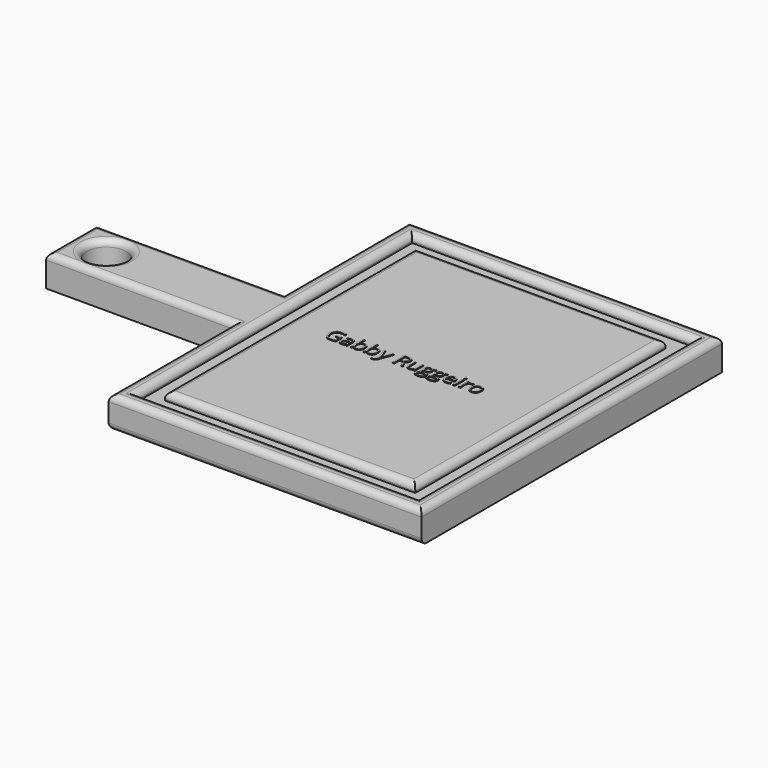
from build123d import *

# Parameters (mm, degrees)
F0_W         = 152.4
F0_H         = 50.8
F1_DEPTH     = 25.4
F2_R         = 15.875
F3_DEPTH     = 25.4
F5_DEPTH     = 6.35
F6_T1_DEPTH  = 228.5999910355
F6_T3_DEPTH  = 279.3999910355
F6_T5_DEPTH  = 330.2
F6_T7_DEPTH  = 279.4
F6_T9_DEPTH  = 139.7
F6_T11_DEPTH = 139.7
F6_T13_DEPTH = 228.5999783039
F6_T15_DEPTH = 279.3999783039
F6_T17_DEPTH = 76.2
F6_T19_DEPTH = 165.1
F6_T27_DEPTH = 292.0999910355
F6_T31_DEPTH = 241.2999910355
F6_T38_DEPTH = 241.2999910355
F6_T42_DEPTH = 292.0999910355
F6_T49_DEPTH = 292.0999910355
F6_T53_DEPTH = 241.2999910355
F6_T60_DEPTH = 292.0999910355
F6_T64_DEPTH = 241.2999910355
F6_T71_DEPTH = 152.4
F6_T75_DEPTH = 177.8
F6_T82_DEPTH = 152.4
F6_T86_DEPTH = 177.8
F7_TEXT_SIZE = 17.0792183232
F8_DEPTH     = 0.508


# Not quite as in the source:
# - a fillet or chamfer that OpenCascade refuses, or shapes differently, is made with other operations: its cross-section is extruded or revolved along the edge and cut away or added
# - Text() gives the source's letters only with a copy of the font that has no kerning and outlines rounded to 1/6400 em; it was checked with that copy


with BuildPart() as f1:
    # F0 (on Top) → F1 (new body)
    with BuildSketch(Plane.XY):
        Polygon((127, -152.4), (127, 152.4), (-127, 152.4), (-127, 25.4), (-127, -25.4), (-127, -152.4), align=None)
        with Locations((-203.2, 0)):
            Rectangle(F0_W, F0_H)
    extrude(amount=F1_DEPTH)

    # F2 (on face) → F3 (cut)
    with BuildSketch(Plane.XY.offset(25.4)):
        with Locations((-250.825, 0)):
            Circle(F2_R)
    extrude(amount=-F3_DEPTH, mode=Mode.SUBTRACT)

    # F4 (on face) → F5 (cut)
    with BuildSketch(Plane.XY.offset(25.4)):
        Polygon((114.2999955177, 139.6999955177), (-114.2999955177, 139.6999955177), (-114.2999955177, 25.4), (-114.2999955177, -25.4), (-114.2999955177, -139.6999955177), (114.2999955177, -139.6999955177), align=None)
        Polygon((-101.599989152, 126.999989152), (101.599989152, 126.999989152), (101.599989152, -126.999989152), (-101.599989152, -126.999989152), (-101.599989152, -25.4), (-101.599989152, 25.4), align=None, mode=Mode.SUBTRACT)
    extrude(amount=-F5_DEPTH, mode=Mode.SUBTRACT)

    # F6: fillet of radius 5.08 on 19 edges, made by hand

    # F6_s2 → F6_t1 (cut)
    with BuildSketch(Plane.YZ.offset(-114.2999955177)):
        with BuildLine():
            ThreePointArc((144.7799955177, 25.4), (141.1878930693, 23.9121024484), (139.6999955177, 20.32))
            Line((139.6999955177, 20.32), (139.6999955177, 25.4))
            Line((139.6999955177, 25.4), (144.7799955177, 25.4))
        make_face()
        with BuildLine():
            ThreePointArc((-144.7799955177, 25.4), (-141.1878930693, 23.9121024484), (-139.6999955177, 20.32))
            Line((-139.6999955177, 20.32), (-139.6999955177, 25.4))
            Line((-139.6999955177, 25.4), (-144.7799955177, 25.4))
        make_face()
    extrude(amount=F6_T1_DEPTH, mode=Mode.SUBTRACT)

    # F6_s4 → F6_t3 (cut)
    with BuildSketch(Plane.XZ.offset(-139.6999955177)):
        with BuildLine():
            ThreePointArc((-119.3799955177, 25.4), (-115.7878930693, 23.9121024484), (-114.2999955177, 20.32))
            Line((-114.2999955177, 20.32), (-114.2999955177, 25.4))
            Line((-114.2999955177, 25.4), (-119.3799955177, 25.4))
        make_face()
        with BuildLine():
            ThreePointArc((119.3799955177, 25.4), (115.7878930693, 23.9121024484), (114.2999955177, 20.32))
            Line((114.2999955177, 20.32), (114.2999955177, 25.4))
            Line((114.2999955177, 25.4), (119.3799955177, 25.4))
        make_face()
    extrude(amount=F6_T3_DEPTH, mode=Mode.SUBTRACT)

    # F6_s6 → F6_t5 (cut)
    with BuildSketch(Plane.XZ.offset(-165.1)):
        with BuildLine():
            ThreePointArc((127, 20.32), (125.5121024484, 23.9121024484), (121.92, 25.4))
            Line((121.92, 25.4), (127, 25.4))
            Line((127, 25.4), (127, 20.32))
        make_face()
    extrude(amount=F6_T5_DEPTH, mode=Mode.SUBTRACT)

    # F6_s8 → F6_t7 (cut)
    with BuildSketch(Plane.YZ.offset(-139.7)):
        with BuildLine():
            ThreePointArc((-152.4, 20.32), (-150.9121024484, 23.9121024484), (-147.32, 25.4))
            Line((-147.32, 25.4), (-152.4, 25.4))
            Line((-152.4, 25.4), (-152.4, 20.32))
        make_face()
        with BuildLine():
            ThreePointArc((152.4, 20.32), (150.9121024484, 23.9121024484), (147.32, 25.4))
            Line((147.32, 25.4), (152.4, 25.4))
            Line((152.4, 25.4), (152.4, 20.32))
        make_face()
        with BuildLine():
            ThreePointArc((-152.4, 5.08), (-150.9121024484, 1.4878975516), (-147.32, 0))
            Line((-147.32, 0), (-152.4, 0))
            Line((-152.4, 0), (-152.4, 5.08))
        make_face()
    extrude(amount=F6_T7_DEPTH, mode=Mode.SUBTRACT)

    # F6_s10 → F6_t9 (cut)
    with BuildSketch(Plane.XZ.offset(25.4)):
        with BuildLine():
            ThreePointArc((-121.92, 25.4), (-125.5121024484, 23.9121024484), (-127, 20.32))
            Line((-127, 20.32), (-127, 25.4))
            Line((-127, 25.4), (-121.92, 25.4))
        make_face()
        with BuildLine():
            ThreePointArc((-121.92, 0), (-125.5121024484, 1.4878975516), (-127, 5.08))
            Line((-127, 5.08), (-127, 0))
            Line((-127, 0), (-121.92, 0))
        make_face()
    extrude(amount=F6_T9_DEPTH, mode=Mode.SUBTRACT)

    # F6_s12 → F6_t11 (cut)
    with BuildSketch(Plane.XZ.offset(-165.1)):
        with BuildLine():
            ThreePointArc((-121.92, 25.4), (-125.5121024484, 23.9121024484), (-127, 20.32))
            Line((-127, 20.32), (-127, 25.4))
            Line((-127, 25.4), (-121.92, 25.4))
        make_face()
    extrude(amount=F6_T11_DEPTH, mode=Mode.SUBTRACT)

    # F6_s14 → F6_t13 (cut)
    with BuildSketch(Plane.YZ.offset(-114.299989152)):
        with BuildLine():
            ThreePointArc((126.999989152, 20.32), (125.5120916004, 23.9121024484), (121.919989152, 25.4))
            Line((121.919989152, 25.4), (126.999989152, 25.4))
            Line((126.999989152, 25.4), (126.999989152, 20.32))
        make_face()
        with BuildLine():
            ThreePointArc((-126.999989152, 20.32), (-125.5120916004, 23.9121024484), (-121.919989152, 25.4))
            Line((-121.919989152, 25.4), (-126.999989152, 25.4))
            Line((-126.999989152, 25.4), (-126.999989152, 20.32))
        make_face()
    extrude(amount=F6_T13_DEPTH, mode=Mode.SUBTRACT)

    # F6_s16 → F6_t15 (cut)
    with BuildSketch(Plane.XZ.offset(-139.699989152)):
        with BuildLine():
            ThreePointArc((101.599989152, 20.32), (100.1120916004, 23.9121024484), (96.519989152, 25.4))
            Line((96.519989152, 25.4), (101.599989152, 25.4))
            Line((101.599989152, 25.4), (101.599989152, 20.32))
        make_face()
        with BuildLine():
            ThreePointArc((-101.599989152, 20.32), (-100.1120916004, 23.9121024484), (-96.519989152, 25.4))
            Line((-96.519989152, 25.4), (-101.599989152, 25.4))
            Line((-101.599989152, 25.4), (-101.599989152, 20.32))
        make_face()
    extrude(amount=F6_T15_DEPTH, mode=Mode.SUBTRACT)

    # F6_s18 → F6_t17 (cut)
    with BuildSketch(Plane.XZ.offset(-38.1)):
        with BuildLine():
            ThreePointArc((-274.32, 25.4), (-277.9121024484, 23.9121024484), (-279.4, 20.32))
            Line((-279.4, 20.32), (-279.4, 25.4))
            Line((-279.4, 25.4), (-274.32, 25.4))
        make_face()
    extrude(amount=F6_T17_DEPTH, mode=Mode.SUBTRACT)

    # F6_s20 → F6_t19 (cut)
    with BuildSketch(Plane.YZ.offset(-292.1)):
        with BuildLine():
            ThreePointArc((20.32, 25.4), (23.9121024484, 23.9121024484), (25.4, 20.32))
            Line((25.4, 20.32), (25.4, 25.4))
            Line((25.4, 25.4), (20.32, 25.4))
        make_face()
        with BuildLine():
            ThreePointArc((-20.32, 25.4), (-23.9121024484, 23.9121024484), (-25.4, 20.32))
            Line((-25.4, 20.32), (-25.4, 25.4))
            Line((-25.4, 25.4), (-20.32, 25.4))
        make_face()
    extrude(amount=F6_T19_DEPTH, mode=Mode.SUBTRACT)

    # F6_s21 → F6_t22 (revolve, cut)
    with BuildSketch(Plane.XZ):
        with BuildLine():
            ThreePointArc((-229.87, 25.4), (-233.4621024484, 23.9121024484), (-234.95, 20.32))
            Line((-234.95, 20.32), (-234.95, 25.4))
            Line((-234.95, 25.4), (-229.87, 25.4))
        make_face()
    revolve(axis=Axis((-250.825, 0, 25.4), (0, 0, 1)), mode=Mode.SUBTRACT)


with BuildPart() as f6_tool25:
    # F6_s26 → F6_t27 (new body)
    with BuildSketch(Plane.XZ.offset(139.6999955177)):
        with BuildLine():
            ThreePointArc((119.3799955177, 25.4), (115.7878930693, 23.9121024484), (114.2999955177, 20.32))
            Line((114.2999955177, 20.32), (114.2999955177, 25.4))
            Line((114.2999955177, 25.4), (119.3799955177, 25.4))
        make_face()
    extrude(amount=-F6_T27_DEPTH)

    split(bisect_by=Plane.XZ.offset(-139.6999955177), keep=Keep.BOTTOM)


with BuildPart() as f6_tool29:
    # F6_s30 → F6_t31 (new body)
    with BuildSketch(Plane.YZ.offset(126.9999955177)):
        with BuildLine():
            ThreePointArc((144.7799955177, 25.4), (141.1878930693, 23.9121024484), (139.6999955177, 20.32))
            Line((139.6999955177, 20.32), (139.6999955177, 25.4))
            Line((139.6999955177, 25.4), (144.7799955177, 25.4))
        make_face()
    extrude(amount=-F6_T31_DEPTH)

    split(bisect_by=Plane.YZ.offset(114.2999955177), keep=Keep.TOP)


with BuildPart() as f6_tool25_1:
    add(f6_tool25.part)

    # F6_t33: intersect F6_tool29
    add(f6_tool29.part, mode=Mode.INTERSECT)


with BuildPart() as f1_1:
    add(f1.part)

    # F6_t23: cut F6_tool25
    add(f6_tool25_1.part, mode=Mode.SUBTRACT)


with BuildPart() as f6_tool36:
    # F6_s37 → F6_t38 (new body)
    with BuildSketch(Plane.YZ.offset(114.2999955177)):
        with BuildLine():
            ThreePointArc((144.7799955177, 25.4), (141.1878930693, 23.9121024484), (139.6999955177, 20.32))
            Line((139.6999955177, 20.32), (139.6999955177, 25.4))
            Line((139.6999955177, 25.4), (144.7799955177, 25.4))
        make_face()
    extrude(amount=-F6_T38_DEPTH)

    split(bisect_by=Plane.YZ.offset(-114.2999955177), keep=Keep.BOTTOM)


with BuildPart() as f6_tool40:
    # F6_s41 → F6_t42 (new body)
    with BuildSketch(Plane.XZ.offset(139.6999955177)):
        with BuildLine():
            ThreePointArc((-119.3799955177, 25.4), (-115.7878930693, 23.9121024484), (-114.2999955177, 20.32))
            Line((-114.2999955177, 20.32), (-114.2999955177, 25.4))
            Line((-114.2999955177, 25.4), (-119.3799955177, 25.4))
        make_face()
    extrude(amount=-F6_T42_DEPTH)

    split(bisect_by=Plane.XZ.offset(-139.6999955177), keep=Keep.BOTTOM)


with BuildPart() as f6_tool36_1:
    add(f6_tool36.part)

    # F6_t44: intersect F6_tool40
    add(f6_tool40.part, mode=Mode.INTERSECT)


with BuildPart() as f1_2:
    add(f1_1.part)

    # F6_t34: cut F6_tool36
    add(f6_tool36_1.part, mode=Mode.SUBTRACT)


with BuildPart() as f6_tool47:
    # F6_s48 → F6_t49 (new body)
    with BuildSketch(Plane.XZ.offset(152.3999955177)):
        with BuildLine():
            ThreePointArc((-119.3799955177, 25.4), (-115.7878930693, 23.9121024484), (-114.2999955177, 20.32))
            Line((-114.2999955177, 20.32), (-114.2999955177, 25.4))
            Line((-114.2999955177, 25.4), (-119.3799955177, 25.4))
        make_face()
    extrude(amount=-F6_T49_DEPTH)

    split(bisect_by=Plane.XZ.offset(139.6999955177), keep=Keep.TOP)


with BuildPart() as f6_tool51:
    # F6_s52 → F6_t53 (new body)
    with BuildSketch(Plane.YZ.offset(-126.9999955177)):
        with BuildLine():
            ThreePointArc((-144.7799955177, 25.4), (-141.1878930693, 23.9121024484), (-139.6999955177, 20.32))
            Line((-139.6999955177, 20.32), (-139.6999955177, 25.4))
            Line((-139.6999955177, 25.4), (-144.7799955177, 25.4))
        make_face()
    extrude(amount=F6_T53_DEPTH)

    split(bisect_by=Plane.YZ.offset(-114.2999955177), keep=Keep.BOTTOM)


with BuildPart() as f6_tool47_1:
    add(f6_tool47.part)

    # F6_t55: intersect F6_tool51
    add(f6_tool51.part, mode=Mode.INTERSECT)


with BuildPart() as f1_3:
    add(f1_2.part)

    # F6_t45: cut F6_tool47
    add(f6_tool47_1.part, mode=Mode.SUBTRACT)


with BuildPart() as f6_tool58:
    # F6_s59 → F6_t60 (new body)
    with BuildSketch(Plane.XZ.offset(152.3999955177)):
        with BuildLine():
            ThreePointArc((119.3799955177, 25.4), (115.7878930693, 23.9121024484), (114.2999955177, 20.32))
            Line((114.2999955177, 20.32), (114.2999955177, 25.4))
            Line((114.2999955177, 25.4), (119.3799955177, 25.4))
        make_face()
    extrude(amount=-F6_T60_DEPTH)

    split(bisect_by=Plane.XZ.offset(139.6999955177), keep=Keep.TOP)


with BuildPart() as f6_tool62:
    # F6_s63 → F6_t64 (new body)
    with BuildSketch(Plane.YZ.offset(-114.2999955177)):
        with BuildLine():
            ThreePointArc((-144.7799955177, 25.4), (-141.1878930693, 23.9121024484), (-139.6999955177, 20.32))
            Line((-139.6999955177, 20.32), (-139.6999955177, 25.4))
            Line((-139.6999955177, 25.4), (-144.7799955177, 25.4))
        make_face()
    extrude(amount=F6_T64_DEPTH)

    split(bisect_by=Plane.YZ.offset(114.2999955177), keep=Keep.TOP)


with BuildPart() as f6_tool58_1:
    add(f6_tool58.part)

    # F6_t66: intersect F6_tool62
    add(f6_tool62.part, mode=Mode.INTERSECT)


with BuildPart() as f1_4:
    add(f1_3.part)

    # F6_t56: cut F6_tool58
    add(f6_tool58_1.part, mode=Mode.SUBTRACT)


with BuildPart() as f6_tool69:
    # F6_s70 → F6_t71 (new body)
    with BuildSketch(Plane.XZ.offset(12.7)):
        with BuildLine():
            ThreePointArc((-121.92, 25.4), (-125.5121024484, 23.9121024484), (-127, 20.32))
            Line((-127, 20.32), (-127, 25.4))
            Line((-127, 25.4), (-121.92, 25.4))
        make_face()
    extrude(amount=F6_T71_DEPTH)

    split(bisect_by=Plane.XZ.offset(25.4), keep=Keep.BOTTOM)


with BuildPart() as f6_tool73:
    # F6_s74 → F6_t75 (new body)
    with BuildSketch(Plane.YZ.offset(-292.1)):
        with BuildLine():
            ThreePointArc((-20.32, 25.4), (-23.9121024484, 23.9121024484), (-25.4, 20.32))
            Line((-25.4, 20.32), (-25.4, 25.4))
            Line((-25.4, 25.4), (-20.32, 25.4))
        make_face()
    extrude(amount=F6_T75_DEPTH)

    split(bisect_by=Plane.YZ.offset(-127), keep=Keep.TOP)


with BuildPart() as f6_tool69_1:
    add(f6_tool69.part)

    # F6_t77: intersect F6_tool73
    add(f6_tool73.part, mode=Mode.INTERSECT)


with BuildPart() as f1_5:
    add(f1_4.part)

    # F6_t67: cut F6_tool69
    add(f6_tool69_1.part, mode=Mode.SUBTRACT)


with BuildPart() as f6_tool80:
    # F6_s81 → F6_t82 (new body)
    with BuildSketch(Plane.XZ.offset(-165.1)):
        with BuildLine():
            ThreePointArc((-121.92, 25.4), (-125.5121024484, 23.9121024484), (-127, 20.32))
            Line((-127, 20.32), (-127, 25.4))
            Line((-127, 25.4), (-121.92, 25.4))
        make_face()
    extrude(amount=F6_T82_DEPTH)

    split(bisect_by=Plane.XZ.offset(-25.4), keep=Keep.TOP)


with BuildPart() as f6_tool84:
    # F6_s85 → F6_t86 (new body)
    with BuildSketch(Plane.YZ.offset(-114.3)):
        with BuildLine():
            ThreePointArc((20.32, 25.4), (23.9121024484, 23.9121024484), (25.4, 20.32))
            Line((25.4, 20.32), (25.4, 25.4))
            Line((25.4, 25.4), (20.32, 25.4))
        make_face()
    extrude(amount=-F6_T86_DEPTH)

    split(bisect_by=Plane.YZ.offset(-127), keep=Keep.TOP)


with BuildPart() as f6_tool80_1:
    add(f6_tool80.part)

    # F6_t88: intersect F6_tool84
    add(f6_tool84.part, mode=Mode.INTERSECT)


with BuildPart() as f1_6:
    add(f1_5.part)

    # F6_t78: cut F6_tool80
    add(f6_tool80_1.part, mode=Mode.SUBTRACT)

    # F7 (on face) → F8 (join)
    with BuildSketch(Plane.XY.offset(25.4)):
        with Locations((-71.119989152, -6.0789489949)):
            Text('Gabby Ruggeiro', F7_TEXT_SIZE, font='Open Sans', text_align=(TextAlign.LEFT, TextAlign.BOTTOM))
    extrude(amount=F8_DEPTH)


solid = f1_6.part
